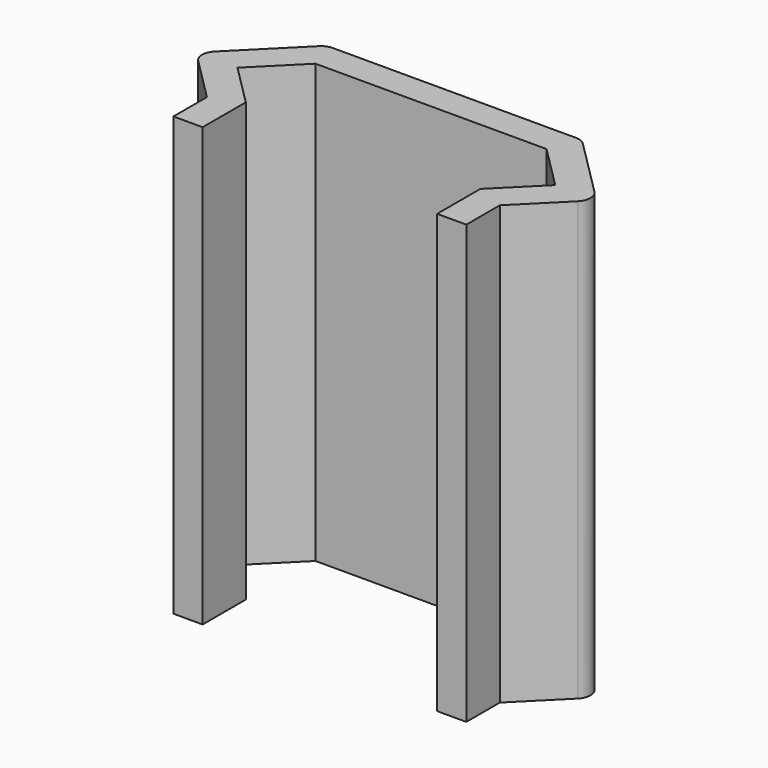
from build123d import *

# Parameters (mm, degrees)
F3_DEPTH     = 30
F4_TEXT_SIZE = 8.5419535792
F5_DEPTH     = 0.5
F6_R         = 1


# Not quite as in the source:
# - Text() gives the source's letters only with a copy of the font that has no kerning and outlines rounded to 1/6400 em; it was checked with that copy


with BuildPart() as f3:
    # F2 (on offset) → F3 (new body)
    with BuildSketch(Plane.XY.offset(10)):
        Polygon((8.035, -2.5161978224), (8.035, -6.2133551099), (10.035, -6.2133551099), (10.035, -3.3446249471), (13.7162698372, 0.3366448901), (8.7462698372, 5.3066448901), (0, 5.3066448901), (-8.7462698372, 5.3066448901), (-13.7162698372, 0.3366448901), (-10.035, -3.3446249471), (-10.035, -6.2133551099), (-8.035, -6.2133551099), (-8.035, -2.5161978224), (-10.8878427125, 0.3366448901), (-7.9178427125, 3.3066448901), (0, 3.3066448901), (7.9178427125, 3.3066448901), (10.8878427125, 0.3366448901), align=None)
    extrude(amount=F3_DEPTH)

    # F4 (on face) → F5 (cut)
    with BuildSketch(Plane(origin=(0, 5.3066448901, 0), x_dir=(-1, 0, 0), z_dir=(0, 1, 0))):
        with Locations(Location((3.0751032885, 11.9988797164), (0, 0, 90))):
            Text('PLEXY', F4_TEXT_SIZE, font='Open Sans', font_style=FontStyle.BOLD, text_align=(TextAlign.LEFT, TextAlign.BOTTOM))
        with BuildLine():
            Line((-1.963314643, 14.0596260174), (-0.1534882284, 14.0596260174))
            Line((-0.1534882284, 14.0596260174), (-0.1534882284, 14.4853890161))
            add(Edge.make_bspline(
                [(-0.1534882284, 14.4853890161), (-0.1534882284, 15.0806564062), (-0.3890592919, 15.376955421)],
                knots=[0, 0, 0, 1, 1, 1], degree=2))
            add(Edge.make_bspline(
                [(-0.3890592919, 15.376955421), (-0.6246303555, 15.6732544357), (-1.0744175986, 15.6732544357)],
                knots=[0, 0, 0, 1, 1, 1], degree=2))
            add(Edge.make_bspline(
                [(-1.0744175986, 15.6732544357), (-1.5295435628, 15.6732544357), (-1.7464291029, 15.4250039098)],
                knots=[0, 0, 0, 1, 1, 1], degree=2))
            add(Edge.make_bspline(
                [(-1.7464291029, 15.4250039098), (-1.963314643, 15.1767533839), (-1.963314643, 14.646885326)],
                knots=[0, 0, 0, 1, 1, 1], degree=2))
            Line((-1.963314643, 14.646885326), (-1.963314643, 14.0596260174))
        make_face()
    extrude(amount=-F5_DEPTH, mode=Mode.SUBTRACT)

    # F6
    f6_edges = [f3.edges().sort_by_distance(p)[0] for p in [
        (-13.71627, 0.336645, 25),
        (-8.74627, 5.306645, 25),
        (8.74627, 5.306645, 25),
        (13.71627, 0.336645, 25),
    ]]
    fillet(f6_edges, radius=F6_R)


solid = f3.part
